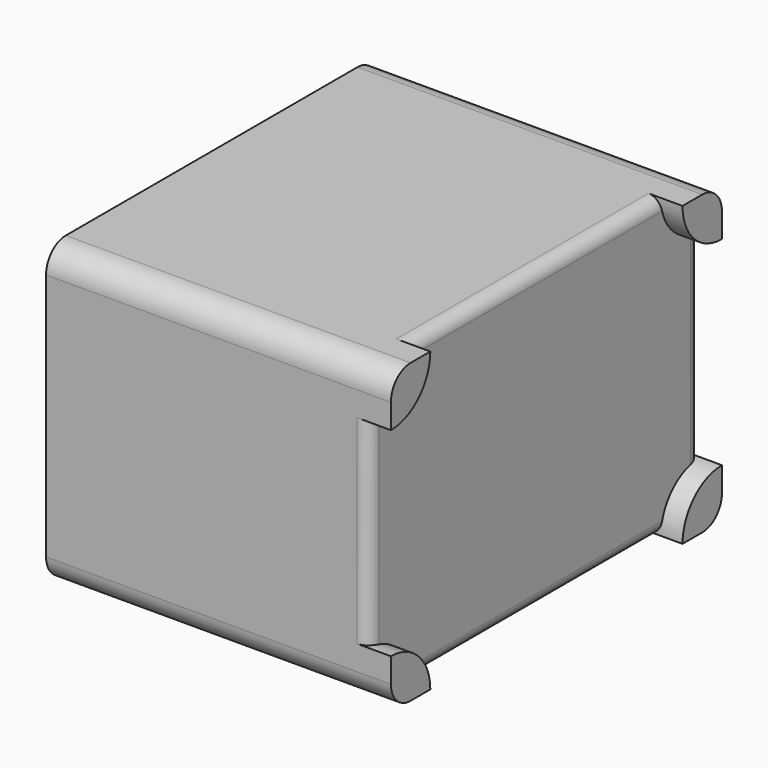
from build123d import *

# Parameters (mm, degrees)
F1_DEPTH = 1.524
F3_DEPTH = 40.132
F5_DEPTH = 2.794
F8_R     = 1.5875
F9_R     = 1.5875
F10_R    = 1.5875
F11_R    = 1.5875


with BuildPart() as f1:
    # F0 (on Right) → F1 (new body)
    with BuildSketch(Plane.YZ):
        with BuildLine():
            ThreePointArc((26.67, 16.002), (25.7400640303, 18.2470640303), (23.495, 19.177))
            Line((23.495, 19.177), (-23.495, 19.177))
            ThreePointArc((-23.495, 19.177), (-25.7400640303, 18.2470640303), (-26.67, 16.002))
            Line((-26.67, 16.002), (-26.67, -16.002))
            ThreePointArc((-26.67, -16.002), (-25.7400640303, -18.2470640303), (-23.495, -19.177))
            Line((-23.495, -19.177), (23.495, -19.177))
            ThreePointArc((23.495, -19.177), (25.7400640303, -18.2470640303), (26.67, -16.002))
            Line((26.67, -16.002), (26.67, 16.002))
        make_face()
    extrude(amount=F1_DEPTH)

    # F2 (on face) → F3 (join)
    with BuildSketch(Plane(origin=(0, 0, 0), x_dir=(0, -1, 0), z_dir=(-1, 0, 0))):
        with BuildLine():
            ThreePointArc((-23.495, 19.177), (-25.7400640303, 18.2470640303), (-26.67, 16.002))
            Line((-26.67, 16.002), (-26.67, -16.002))
            ThreePointArc((-26.67, -16.002), (-25.7400640303, -18.2470640303), (-23.495, -19.177))
            Line((-23.495, -19.177), (23.495, -19.177))
            ThreePointArc((23.495, -19.177), (25.7400640303, -18.2470640303), (26.67, -16.002))
            Line((26.67, -16.002), (26.67, 16.002))
            ThreePointArc((26.67, 16.002), (25.7400640303, 18.2470640303), (23.495, 19.177))
            Line((23.495, 19.177), (-23.495, 19.177))
        make_face()
        with BuildLine():
            ThreePointArc((25.146, -16.0655), (24.6810320151, -17.1880320151), (23.5585, -17.653))
            Line((23.5585, -17.653), (-23.5585, -17.653))
            ThreePointArc((-23.5585, -17.653), (-24.6810320151, -17.1880320151), (-25.146, -16.0655))
            Line((-25.146, -16.0655), (-25.146, 16.0655))
            ThreePointArc((-25.146, 16.0655), (-24.6810320151, 17.1880320151), (-23.5585, 17.653))
            Line((-23.5585, 17.653), (23.5585, 17.653))
            ThreePointArc((23.5585, 17.653), (24.6810320151, 17.1880320151), (25.146, 16.0655))
            Line((25.146, 16.0655), (25.146, -16.0655))
        make_face(mode=Mode.SUBTRACT)
    extrude(amount=F3_DEPTH)

    # F4 (on face) → F5 (join)
    with BuildSketch(Plane.YZ.offset(1.524)):
        with BuildLine():
            ThreePointArc((-26.67, 12.827), (-22.1798719395, 14.6868719395), (-20.32, 19.177))
            Line((-20.32, 19.177), (-23.495, 19.177))
            ThreePointArc((-23.495, 19.177), (-25.7400640303, 18.2470640303), (-26.67, 16.002))
            Line((-26.67, 16.002), (-26.67, 12.827))
        make_face()
    extrude(amount=F5_DEPTH)


with BuildPart() as f6_1:
    # F6: instance of F1
    add(f1.part.mirror(Plane.XY))


with BuildPart() as f1_1:
    add(f1.part)

    add(f6_1.part)  # F7 merges F6_1
    # F7: F6_1, F1 across plane
    add(f6_1.part.mirror(Plane.XZ))
    add(f1.part.mirror(Plane.XZ))

    # F8
    f8_edges = [f1_1.edges().sort_by_distance(p)[0] for p in [
        (1.524, -26.67, 0),
    ]]
    fillet(f8_edges, radius=F8_R)

    # F9
    f9_edges = [f1_1.edges().sort_by_distance(p)[0] for p in [
        (1.524, 0, -19.177),
    ]]
    fillet(f9_edges, radius=F9_R)

    # F10
    f10_edges = [f1_1.edges().sort_by_distance(p)[0] for p in [
        (1.524, 26.67, 0),
    ]]
    fillet(f10_edges, radius=F10_R)

    # F11
    f11_edges = [f1_1.edges().sort_by_distance(p)[0] for p in [
        (1.524, 0, 19.177),
    ]]
    fillet(f11_edges, radius=F11_R)


solid = f1_1.part
